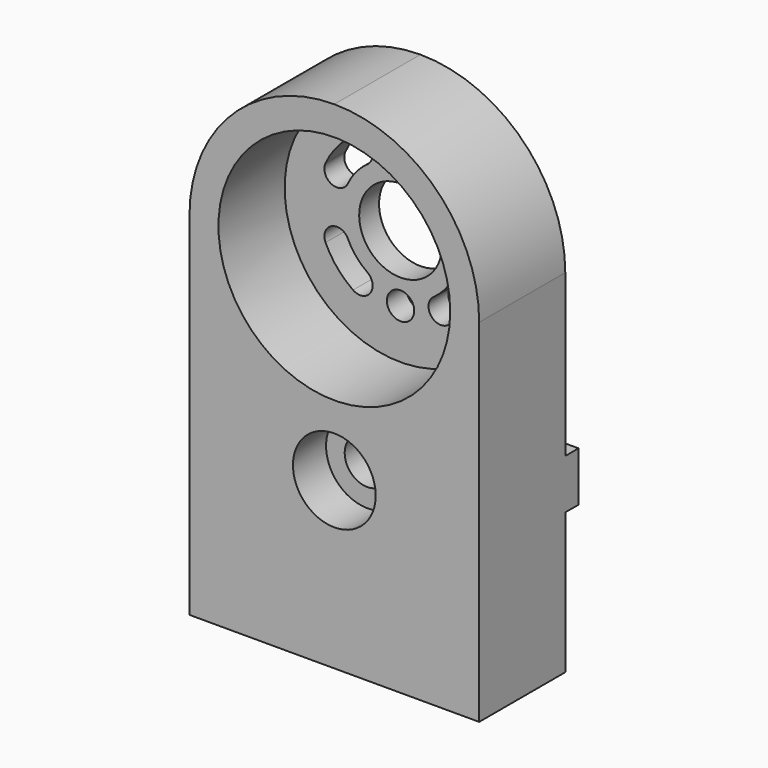
from build123d import *

# Parameters (mm, degrees)
F0_W             = 35
F0_H             = 60
F1_DEPTH         = 15
F2_R             = 5
F3_DEPTH         = 25
F4_T1_DEPTH      = 102.5
F6_DEPTH         = 15.001
F6_COPIES2_COUNT = 2
F8_R             = 14
F9_DEPTH         = 10
F10_W            = 35
F10_H            = 17
F11_DEPTH        = 2
F13_D            = 5.5
F13_CBORE_D      = 10
F13_CBORE_DEPTH  = 5
F15_D            = 3.3


# Not quite as in the source:
# - a fillet or chamfer that OpenCascade refuses, or shapes differently, is made with other operations: its cross-section is extruded or revolved along the edge and cut away or added
# - a pattern or mirror of a feature is missing from the dataset's text; its kind, count and spacing are read off the source's solid


with BuildPart() as f1:
    # F0 (on Front) → F1 (new body)
    with BuildSketch(Plane.XZ):
        Rectangle(F0_W, F0_H)
    extrude(amount=F1_DEPTH)

    # F2 (on face) → F3 (cut)
    with BuildSketch(Plane(origin=(0, 0, 0), x_dir=(-1, 0, 0), z_dir=(0, 1, 0))):
        with Locations((0, 12.5)):
            Circle(F2_R)
    extrude(amount=-F3_DEPTH, mode=Mode.SUBTRACT)

    # F4: fillet of radius 17.5 on 2 edges, made by hand

    # F4_s2 → F4_t1 (cut)
    with BuildSketch(Plane.XZ.offset(-43.75)):
        with BuildLine():
            ThreePointArc((0, 30), (12.3743686708, 24.8743686708), (17.5, 12.5))
            Line((17.5, 12.5), (17.5, 30))
            Line((17.5, 30), (0, 30))
        make_face()
        with BuildLine():
            ThreePointArc((0, 30), (-12.3743686708, 24.8743686708), (-17.5, 12.5))
            Line((-17.5, 12.5), (-17.5, 30))
            Line((-17.5, 30), (0, 30))
        make_face()
    extrude(amount=F4_T1_DEPTH, mode=Mode.SUBTRACT)

    # F5 (on face) → F6 (cut, through all)
    with BuildSketch(Plane(origin=(0, 0, 0), x_dir=(-1, 0, 0), z_dir=(0, 1, 0))):
        with BuildLine():
            ThreePointArc((6.3441819771, 15.4582689266), (8.3375643136, 14.73271613), (9.0631171101, 16.7260984665))
            ThreePointArc((9.0631171101, 16.7260984665), (7.6604742725, 18.9278405332), (5.7357643635, 20.6915204429))
            ThreePointArc((5.7357643635, 20.6915204429), (3.6466716426, 20.323157031), (4.0150350545, 18.23406431))
            ThreePointArc((4.0150350545, 18.23406431), (5.3623319908, 16.9994883732), (6.3441819771, 15.4582689266))
        make_face()
    f6 = extrude(amount=-F6_DEPTH, mode=Mode.SUBTRACT)

    # F6_copies: F6 across plane
    add(f6.mirror(Plane(origin=(0, 0, 12.5), x_dir=(-1, 0, 0), z_dir=(0, 0, -1))), mode=Mode.SUBTRACT)

    # F6_copies1: F6 across plane
    add(f6.mirror(Plane(origin=(0, 0, 0), x_dir=(0, 0, 1), z_dir=(1, 0, 0))), mode=Mode.SUBTRACT)

    # F6_copies2: F6 ×2 about axis
    f6_copies2_axis = Axis((0, 0, 12.5), (0, 1, 0))
    for i in range(1, F6_COPIES2_COUNT):
        add(f6.rotate(f6_copies2_axis, i * 360 / F6_COPIES2_COUNT), mode=Mode.SUBTRACT)

    # F8 (on face) → F9 (cut)
    with BuildSketch(Plane.XZ.offset(15)):
        with Locations((0, 12.5)):
            Circle(F8_R)
    extrude(amount=-F9_DEPTH, mode=Mode.SUBTRACT)

    # F10 (on Front) → F11 (cut)
    with BuildSketch(Plane.XZ):
        with BuildLine():
            ThreePointArc((17.5, 12.5), (0, 30), (-17.5, 12.5))
            Line((-17.5, 12.5), (-17.5, -7))
            Line((-17.5, -7), (17.5, -7))
            Line((17.5, -7), (17.5, 12.5))
        make_face()
        with Locations((0, -21.5)):
            Rectangle(F10_W, F10_H)
    extrude(amount=F11_DEPTH, mode=Mode.SUBTRACT)

    # F13 (through all)
    with Locations(Plane.XZ.offset(15)):
        with Locations((0, -10)):
            CounterBoreHole(F13_D / 2, F13_CBORE_D / 2, F13_CBORE_DEPTH)

    # F15 (through all)
    with Locations(Plane(origin=(0, -2, 0), x_dir=(-1, 0, 0), z_dir=(0, 1, 0))):
        with Locations((0, 20.5), (0, 4.5)):
            Hole(F15_D / 2)


solid = f1.part
